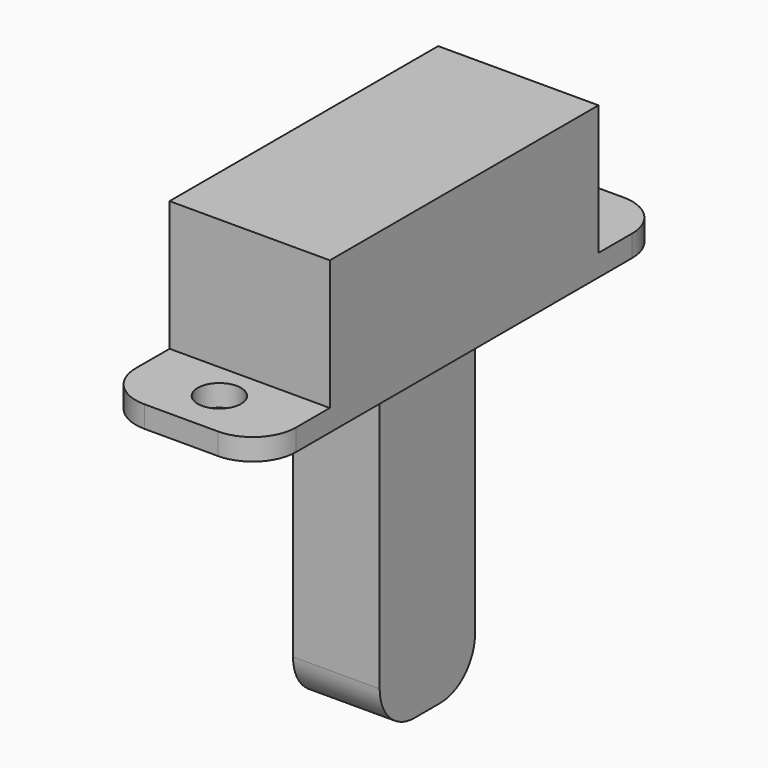
from build123d import *

# Parameters (mm, degrees)
F0_W     = 4
F0_H     = 5.5
F1_DEPTH = 16
F0_W_2   = 7.4
F0_H_2   = 15.5
F0_W_3   = 4.1
F0_H_3   = 8.5
F0_H_4   = 3.95
F0_R     = 1
F2_DEPTH = 1
F3_R     = 2
F4_DEPTH = 6
F5_R     = 2


with BuildPart() as f1:
    # F0 (on Top) → F1 (new body)
    with BuildSketch(Plane.XY):
        Rectangle(F0_W, F0_H)
    extrude(amount=-F1_DEPTH)

    # F5
    f5_edges = [f1.edges().sort_by_distance(p)[0] for p in [
        (0, 2.75, -16),
        (0, -2.75, -16),
    ]]
    fillet(f5_edges, radius=F5_R)


with BuildPart() as f2:
    # F0 (on Top) → F2 (new body)
    with BuildSketch(Plane.XY):
        Rectangle(F0_W_2, F0_H_2)
        Rectangle(F0_W_3, F0_H_3, mode=Mode.SUBTRACT)
        with Locations((0, -9.725)):
            Rectangle(F0_W_2, F0_H_4)
        with Locations((0, -9.5)):
            Circle(F0_R, mode=Mode.SUBTRACT)
        with Locations((0, 9.725)):
            Rectangle(F0_W_2, F0_H_4)
        with Locations((0, 9.5)):
            Circle(F0_R, mode=Mode.SUBTRACT)
    extrude(amount=-F2_DEPTH)

    # F3
    f3_edges = [f2.edges().sort_by_distance(p)[0] for p in [
        (3.7, 11.7, -0.5),
        (-3.7, 11.7, -0.5),
        (3.7, -11.7, -0.5),
        (-3.7, -11.7, -0.5),
    ]]
    fillet(f3_edges, radius=F3_R)

    # F0 (on Top) → F4 (join)
    with BuildSketch(Plane.XY):
        Rectangle(F0_W_2, F0_H_2)
        Rectangle(F0_W_3, F0_H_3, mode=Mode.SUBTRACT)
        Rectangle(F0_W_3, F0_H_3)
        Rectangle(F0_W, F0_H, mode=Mode.SUBTRACT)
        Rectangle(F0_W, F0_H)
    extrude(amount=F4_DEPTH)


solid = Compound([f1.part, f2.part])
